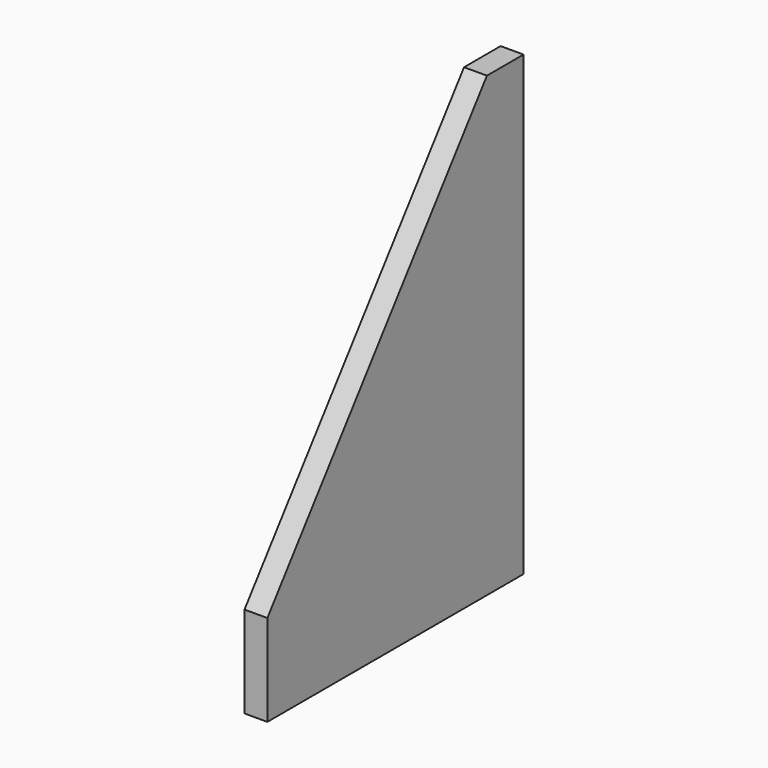
from build123d import *

# Parameters (mm, degrees)
F0_W     = 5
F0_H     = 100
F1_DEPTH = 75
F3_DEPTH = 5
F4_DEPTH = 5


with BuildPart() as f1:
    # F0 (on Front) → F1 (new body)
    with BuildSketch(Plane.XZ):
        with Locations((2.5, 50)):
            Rectangle(F0_W, F0_H)
    extrude(amount=F1_DEPTH)

    # F2 (on face) → F3 (cut)
    with BuildSketch(Plane(origin=(0, 0, 0), x_dir=(0, -1, 0), z_dir=(-1, 0, 0))):
        Polygon((75, 100), (15, 100), (75, 20), align=None)
    extrude(amount=-F3_DEPTH, mode=Mode.SUBTRACT)

    # F4 (cut): a face of the model
    f4_faces = [f1.faces().sort_by_distance(p)[0] for p in [
        (2.5, 0, 50),
    ]]
    extrude(f4_faces, amount=-F4_DEPTH, mode=Mode.SUBTRACT)


solid = f1.part
